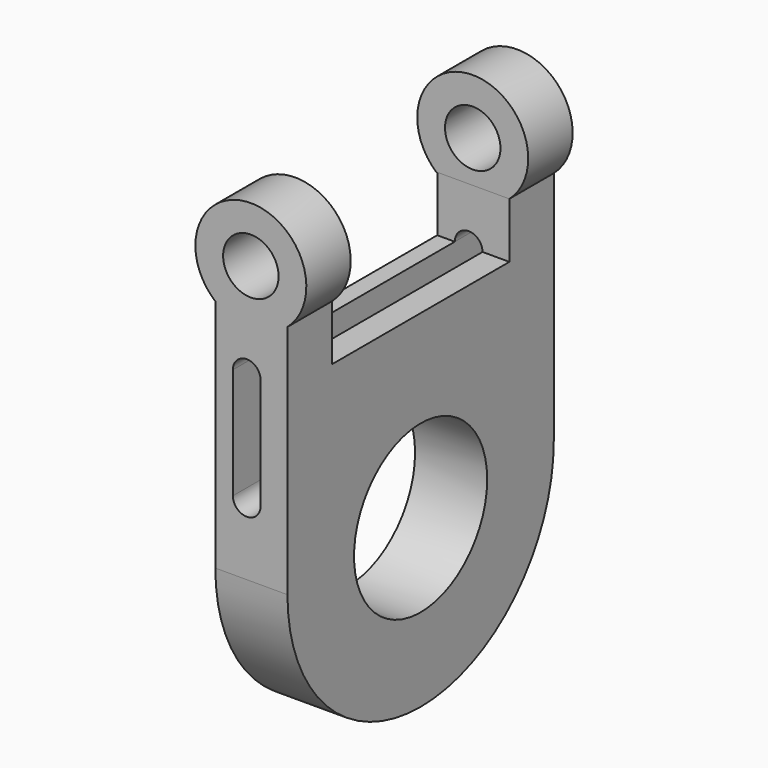
from build123d import *

# Parameters (mm, degrees)
F0_R     = 12.7
F1_DEPTH = 152.4
F2_R     = 76.19999
F3_R     = 38.1
F4_DEPTH = 42.1602994648
F3_W     = 101.6
F3_H     = 25.4
F5_DEPTH = 42.1602994648
F7_DEPTH = 45.29165
F9_DEPTH = 152.401


# Not quite as in the source:
# - a fillet or chamfer is up to 0.001 mm smaller than in the source, because OpenCascade refuses the exact size


with BuildPart() as f1:
    # F0 (on Front) → F1 (new body)
    with BuildSketch(Plane.XZ):
        with BuildLine():
            ThreePointArc((12.2889600906, 43.2626888076), (-4.7984134102, 87.7468446554), (-20.7310399094, 42.83615698))
            Line((-20.7310399094, 42.83615698), (-20.7310399094, -140.8510365048))
            Line((-20.7310399094, -140.8510365048), (12.2889600906, -140.8510365048))
            Line((12.2889600906, -140.8510365048), (12.2889600906, 43.2626888076))
        make_face()
        with Locations((-4.4703393742, 62.3489634952)):
            Circle(F0_R, mode=Mode.SUBTRACT)
    extrude(amount=F1_DEPTH)

    # F2 (radius 76.2 in the source; OpenCascade refuses exactly that, so slightly less here)
    f2_edges = [f1.edges().sort_by_distance(p)[0] for p in [
        (-4.22104, -152.4, -140.851037),
        (-4.22104, 0, -140.851037),
    ]]
    fillet(f2_edges, radius=F2_R)

    # F3 (on face) → F4 (cut, through all)
    with BuildSketch(Plane.YZ.offset(12.2889600906)):
        with Locations((-76.2, -64.6510365048)):
            Circle(F3_R)
    extrude(amount=-F4_DEPTH, mode=Mode.SUBTRACT)

    # F3 (on face) → F5 (cut, through all)
    with BuildSketch(Plane.YZ.offset(12.2889600906)):
        with Locations((-76.2, 30.5626888076)):
            Rectangle(F3_W, F3_H)
    extrude(amount=-F5_DEPTH, mode=Mode.SUBTRACT)

    # F6 (on face) → F7 (cut, symmetric)
    with BuildSketch(Plane(origin=(-20.7310399094, 0, 0), x_dir=(0, -1, 0), z_dir=(-1, 0, 0))):
        Polygon((25.4293922335, 17.8626888076), (127, 17.8626888076), (127, 42.83615698), (127, 109.7837612033), (25.4293922335, 109.7837612033), align=None)
    extrude(amount=F7_DEPTH, both=True, mode=Mode.SUBTRACT)

    # F8 (on face) → F9 (cut, through all)
    with BuildSketch(Plane.XZ.offset(152.4)):
        with BuildLine():
            Line((0, -32.9373111924), (0, 17.8626878918))
            ThreePointArc((0, 17.8626878918), (-6.35, 24.2126888076), (-12.7, 17.8626878918))
            Line((-12.7, 17.8626878918), (-12.7, -32.9373111924))
            ThreePointArc((-12.7, -32.9373111924), (-6.35, -39.2873111924), (0, -32.9373111924))
        make_face()
    extrude(amount=-F9_DEPTH, mode=Mode.SUBTRACT)


solid = f1.part
